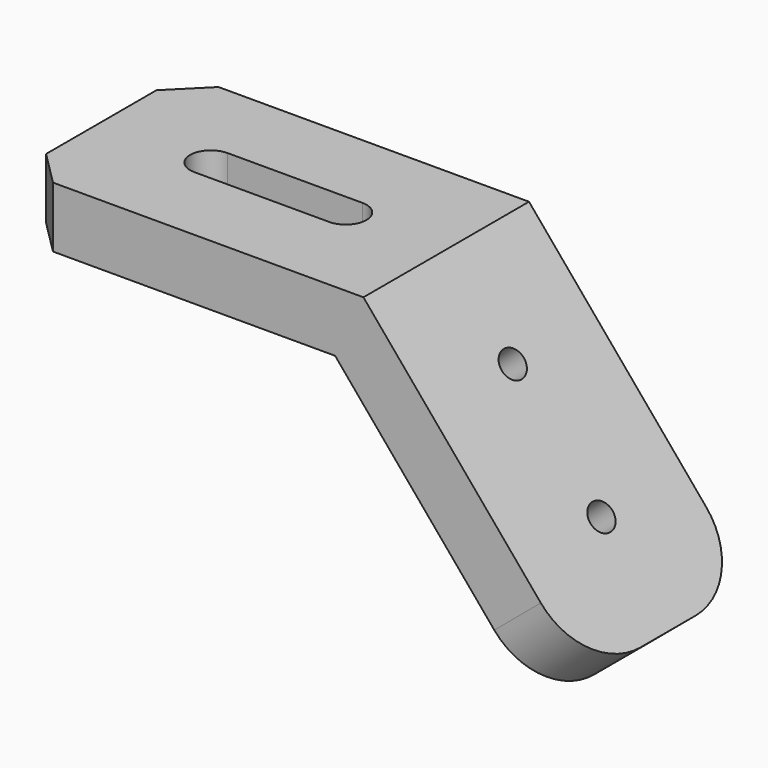
from build123d import *

# Parameters (mm, degrees)
F1_DEPTH = 15
F3_DEPTH = 43.9597531212
F5_D     = 4
F6_R     = 10
F7_SIZE  = 5


with BuildPart() as f1:
    # F0 (on Front) → F1 (new body, symmetric)
    with BuildSketch(Plane.XZ):
        Polygon((50, 0), (0, 0), (0, -8.8), (45.8964926082, -8.8), (75.3981893849, -43.9587531212), (82.1393804843, -38.3022221559), align=None)
    extrude(amount=F1_DEPTH, both=True)

    # F2 (on face) → F3 (cut, through all)
    with BuildSketch(Plane.XY):
        with BuildLine():
            ThreePointArc((15.8875472844, 3), (12.8875472844, 0), (15.8875472844, -3))
            Line((15.8875472844, -3), (35.4375839233, -3))
            ThreePointArc((35.4375839233, -3), (38.4375839233, 0), (35.4375839233, 3))
            Line((35.4375839233, 3), (15.8875472844, 3))
        make_face()
    extrude(amount=-F3_DEPTH, mode=Mode.SUBTRACT)

    # F5 (through all)
    with Locations(Plane(origin=(29.3412044417, 0, 24.6201938253), x_dir=(0, 1, 0), z_dir=(0.7660444431, 0, 0.6427876097))):
        with Locations((0, -47.1393804843), (0, -67.1393804843)):
            Hole(F5_D / 2)

    # F6
    f6_edges = [f1.edges().sort_by_distance(p)[0] for p in [
        (78.768785, -15, -41.130488),
        (78.768785, 15, -41.130488),
    ]]
    fillet(f6_edges, radius=F6_R)

    # F7
    f7_edges = [f1.edges().sort_by_distance(p)[0] for p in [
        (0, -15, -4.4),
        (0, 15, -4.4),
    ]]
    chamfer(f7_edges, length=F7_SIZE)


solid = f1.part
